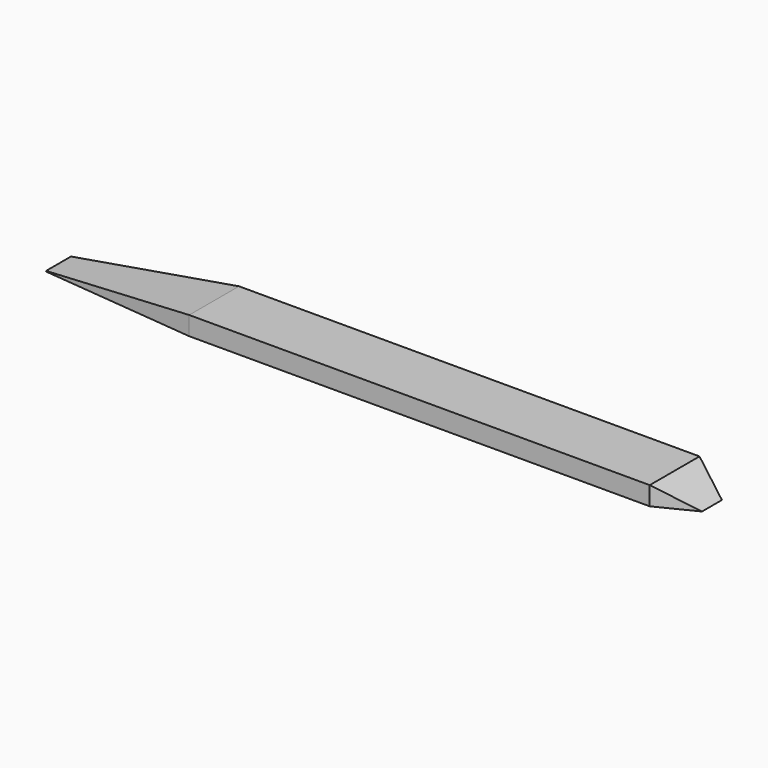
from build123d import *

# Parameters (mm, degrees)
F0_W      = 80
F0_H      = 10
F1_DEPTH  = 3
F1_FACE_W = 10
F1_FACE_H = 3
F3_W      = 5
F3_H      = 0.1
F5_SIZE2  = 5.99999
F5_SIZE   = 2.99999


# Not quite as in the source:
# - a fillet or chamfer is up to 0.001 mm smaller than in the source, because OpenCascade refuses the exact size


with BuildPart() as f1:
    # F0 (on Top) → F1 (new body)
    with BuildSketch(Plane.XY):
        with Locations((0, 5)):
            Rectangle(F0_W, F0_H)
    extrude(amount=F1_DEPTH)

    # F1_face (on face) → F4 section 0
    with BuildSketch(Plane(origin=(-40, 5, 1.5), x_dir=(0, -1, 0), z_dir=(-1, 0, 0))):
        Rectangle(F1_FACE_W, F1_FACE_H)
    # F3 (on plane+point) → F4 section 1
    with BuildSketch(Plane.YZ.offset(-65)):
        with Locations((5, 0.05)):
            Rectangle(F3_W, F3_H)
    loft()

    # F5 (size 3 and 6 in the source; OpenCascade refuses exactly that, so slightly less here)
    f5_edges = [f1.edges().sort_by_distance(p)[0] for p in [
        (40, 5, 3),
        (40, 0, 1.5),
        (40, 10, 1.5),
    ]]
    f5_side = f1.faces().sort_by_distance((40, 5, 1.5))[0]
    chamfer(f5_edges, length=F5_SIZE, length2=F5_SIZE2, reference=f5_side)


solid = f1.part
